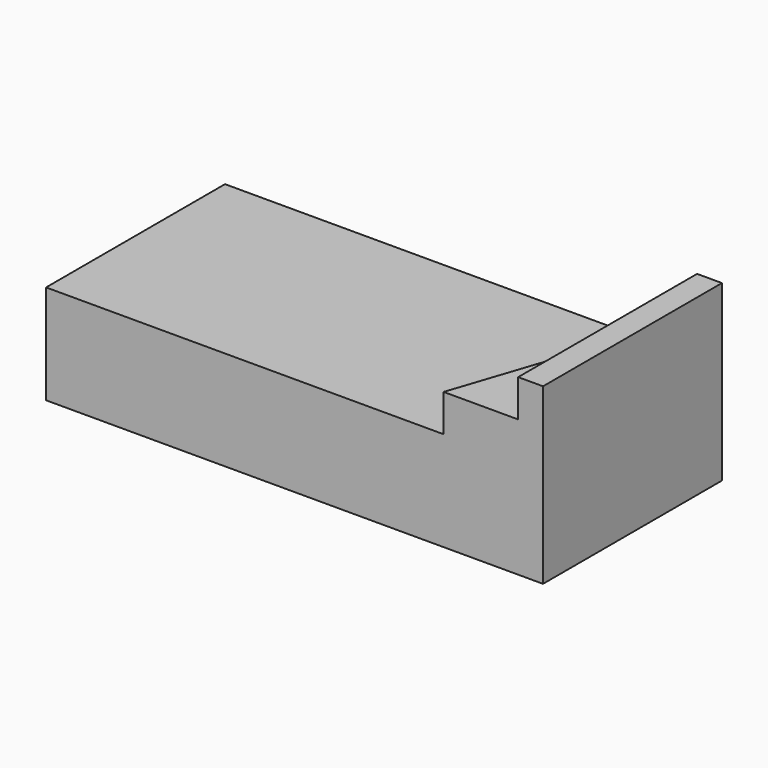
from build123d import *

# Parameters (mm, degrees)
F2_DEPTH = 400
F3_DEPTH = 550
F0_W     = 100
F0_H     = 900
F4_DEPTH = 700


# Not quite as in the source:
# - the program builds the solid bodies; features that only make, move or delete a surface that nothing else refers to are left out


with BuildPart() as f2:
    # F0 (on Top) → F2 (new body)
    with BuildSketch(Plane.XY):
        Polygon((2869.0189361572, -358.3241462708), (969.0189361572, -358.3241462708), (969.0189361572, -1258.3241462708), (2569.0189361572, -1258.3241462708), align=None)
    extrude(amount=F2_DEPTH)

    # F0 (on Top) → F3 (join)
    with BuildSketch(Plane.XY):
        Polygon((2869.0189361572, -1258.3241462708), (2869.0189361572, -358.3241462708), (2569.0189361572, -1258.3241462708), align=None)
    extrude(amount=F3_DEPTH)

    # F0 (on Top) → F4 (join)
    with BuildSketch(Plane.XY):
        with Locations((2919.0189361572, -808.3241462708)):
            Rectangle(F0_W, F0_H)
    extrude(amount=F4_DEPTH)


solid = f2.part
